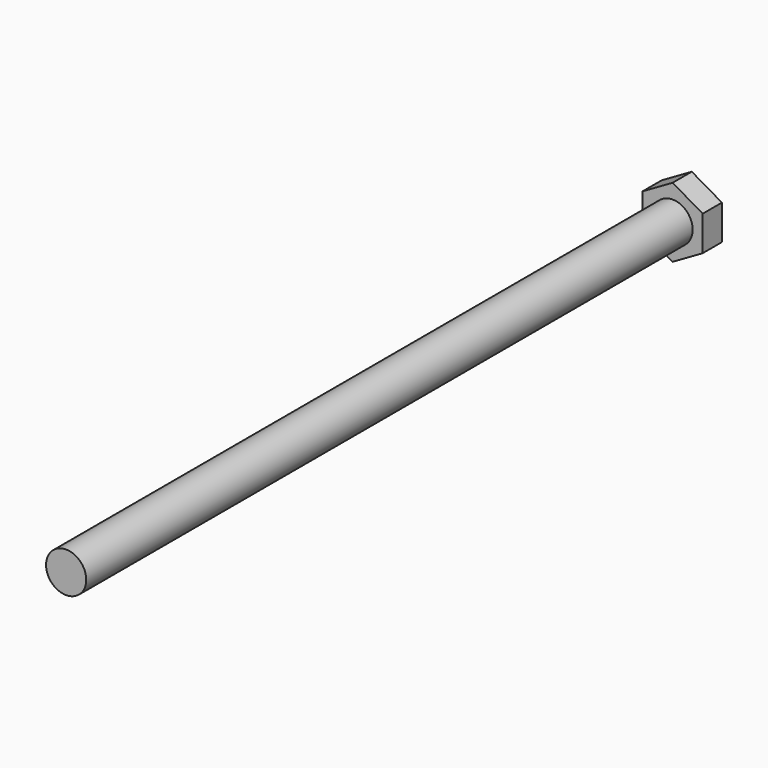
from build123d import *

# Parameters (mm, degrees)
F0_R     = 4.7625
F1_DEPTH = 185.33872
F2_DEPTH = 5.6865671642


# Not quite as in the source:
# - a length typed as a fraction of an inch, garbled in the dataset ("3 / 203.2 mm" for 3/8 in), is restored


with BuildPart() as f1:
    # F0 (on Front) → F1 (new body)
    with BuildSketch(Plane.XZ):
        Circle(F0_R)
    extrude(amount=F1_DEPTH)

    # F0 (on Front) → F2 (join)
    with BuildSketch(Plane.XZ):
        Polygon((7.14375, -4.1244459855), (7.14375, 4.1244459855), (0, 8.248891971), (-7.14375, 4.1244459855), (-7.14375, -4.1244459855), (0, -8.248891971), align=None)
        Circle(F0_R, mode=Mode.SUBTRACT)
    extrude(amount=F2_DEPTH)


solid = f1.part
